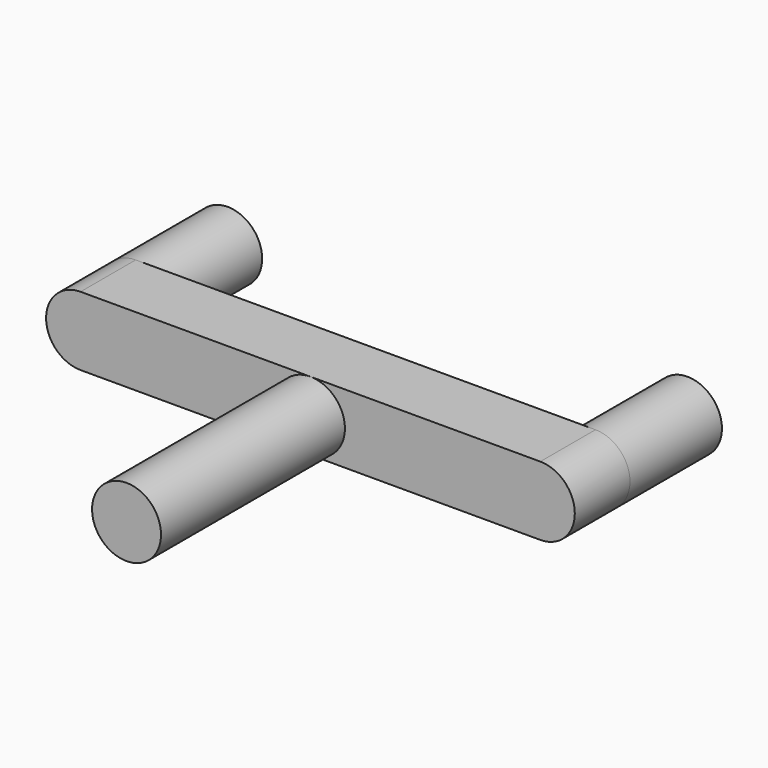
from build123d import *

# Parameters (mm, degrees)
F1_DEPTH = 30
F3_DEPTH = 100
F5_DEPTH = 50


with BuildPart() as f1:
    # F0 (on Front) → F1 (new body)
    with BuildSketch(Plane.XZ):
        with BuildLine():
            Line((100, 15), (-100, 15))
            ThreePointArc((-100, 15), (-115, 0), (-100, -15))
            Line((-100, -15), (100, -15))
            ThreePointArc((100, -15), (115, 0), (100, 15))
        make_face()
    extrude(amount=F1_DEPTH)

    # F2 (on face) → F3 (join)
    with BuildSketch(Plane.XZ.offset(30)):
        with BuildLine():
            ThreePointArc((3.16e-08, -15), (10.606601729, -10.6066017066), (15, 0))
            ThreePointArc((15, 0), (10.6066017178, 10.6066017178), (0, 15))
            ThreePointArc((0, 15), (-15, -1.58e-08), (3.16e-08, -15))
        make_face()
    extrude(amount=F3_DEPTH)

    # F4 (on face) → F5 (join)
    with BuildSketch(Plane(origin=(0, 0, 0), x_dir=(-1, 0, 0), z_dir=(0, 1, 0))):
        with BuildLine():
            ThreePointArc((-100, -15), (-89.3933982822, -10.6066017178), (-85, 0))
            ThreePointArc((-85, 0), (-89.3933982822, 10.6066017178), (-100, 15))
            ThreePointArc((-100, 15), (-115, 0), (-100, -15))
        make_face()
        with BuildLine():
            ThreePointArc((100, 15), (89.3933982822, 10.6066017178), (85, 0))
            ThreePointArc((85, 0), (89.3933982822, -10.6066017178), (100, -15))
            ThreePointArc((100, -15), (110.6066017178, -10.6066017178), (115, 0))
            ThreePointArc((115, 0), (110.6066017178, 10.6066017178), (100, 15))
        make_face()
    extrude(amount=F5_DEPTH)


solid = f1.part
